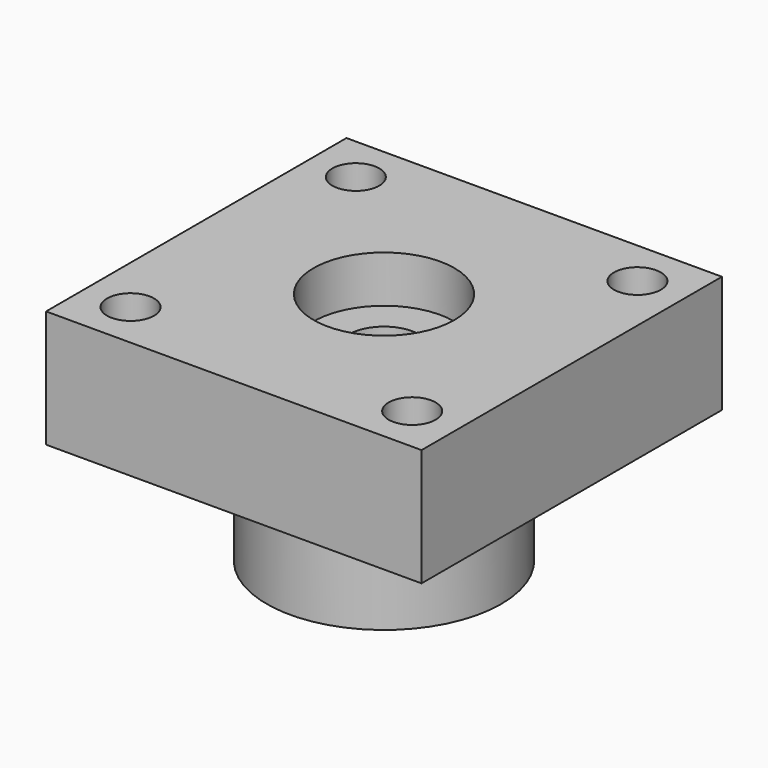
from build123d import *

# Parameters (mm, degrees)
F0_R     = 15
F0_R_2   = 7.5
F1_DEPTH = 15
F2_W     = 80
F2_H     = 80
F2_R     = 5
F2_R_2   = 15
F3_DEPTH = 25
F4_R     = 25
F4_R_2   = 7.5
F5_DEPTH = 25


# Not quite as in the source:
# - a feature names something its author has since deleted; it is built from what else it names


with BuildPart() as f1:
    # F0 (on Top) → F1 (new body)
    with BuildSketch(Plane.XY):
        with Locations((-5.5696061254, -1.9551310688)):
            Circle(F0_R)
        with Locations((-5.5696061254, -1.9551310688)):
            Circle(F0_R_2, mode=Mode.SUBTRACT)
    extrude(amount=F1_DEPTH)


with BuildPart() as f3:
    # F2 (on face) → F3 (new body)
    with BuildSketch(Plane(origin=(0, 0, 0), x_dir=(1, 0, 0), z_dir=(0, 0, -1))):
        with Locations((-5.5696061254, 1.9551310688)):
            Rectangle(F2_W, F2_H)
        with Locations((-35.5696061254, -28.0448689312)):
            Circle(F2_R, mode=Mode.SUBTRACT)
        with Locations((24.4303938746, -28.0448689312)):
            Circle(F2_R, mode=Mode.SUBTRACT)
        with Locations((-35.5696061254, 31.9551310688)):
            Circle(F2_R, mode=Mode.SUBTRACT)
        with Locations((-5.5696061254, 1.9551310688)):
            Circle(F2_R_2, mode=Mode.SUBTRACT)
        with Locations((24.4303938746, 31.9551310688)):
            Circle(F2_R, mode=Mode.SUBTRACT)
    extrude(amount=-F3_DEPTH)


with BuildPart() as f5:
    # F4 (on face) → F5 (new body)
    with BuildSketch(Plane(origin=(0, 0, 0), x_dir=(1, 0, 0), z_dir=(0, 0, -1))):
        with Locations((-5.5696061254, 1.9551310688)):
            Circle(F4_R)
        with Locations((-5.5696061254, 1.9551310688)):
            Circle(F4_R_2, mode=Mode.SUBTRACT)
    extrude(amount=F5_DEPTH)


solid = Compound([f1.part, f3.part, f5.part])
